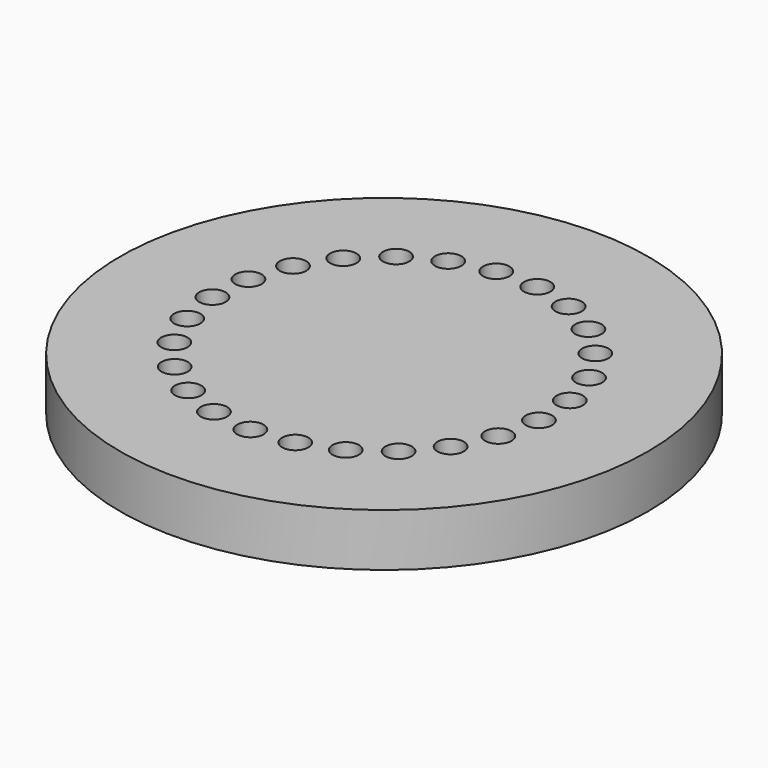
from build123d import *

# Parameters (mm, degrees)
F0_R     = 5080
F1_DEPTH = 508


# Not quite as in the source:
# - a feature names something its author has since deleted; it is built from what else it names


with BuildPart() as f1:
    # F0 (on Top) → F1 (new body, symmetric)
    with BuildSketch(Plane.XY):
        Circle(F0_R)
        with BuildLine():
            ThreePointArc((3159.7651539423, 310.6592537359), (3170.6487728458, 166.1666610714), (3174.9283642102, 21.3279659893))
            ThreePointArc((3174.9283642102, 21.3279659892), (3349.0433755669, -55.9407103788), (3420.4734651877, -232.5312758802))
            ThreePointArc((3420.4734651877, -232.5312758802), (3335.6199052673, -422.018694482), (3137.7531359879, -484.902317584))
            ThreePointArc((3137.7531359879, -484.902317584), (3112.360979424, -627.5620557037), (3080.486200819, -768.9146679337))
            ThreePointArc((3080.486200819, -768.9146679337), (3212.4276604766, -860.3797880933), (3263.1647017804, -1012.6958070214))
            ThreePointArc((3263.1647017804, -1012.6958070214), (3153.2283007654, -1221.8887310114), (2918.5845486504, -1249.9956929441))
            ThreePointArc((2918.5845486504, -1249.9956929442), (2858.512099202, -1381.8587405071), (2792.4857601946, -1510.8435653999))
            ThreePointArc((2792.4857601946, -1510.8435654), (2883.5294819577, -1603.5895784257), (2916.7790532267, -1729.2289361727))
            ThreePointArc((2916.7790532267, -1729.2289361727), (2779.4878421015, -1954.8282681739), (2516.0305603182, -1936.547241754))
            ThreePointArc((2516.0305603182, -1936.5472417539), (2425.052390915, -2049.3281585235), (2329.0231692129, -2157.8406051582))
            ThreePointArc((2329.0231692129, -2157.8406051582), (2383.8377363773, -2240.1269627642), (2403.0812037424, -2337.1082516052))
            ThreePointArc((2403.0812037424, -2337.1082516052), (2236.5946151881, -2575.5561553853), (1955.385118568, -2501.4184052418))
            ThreePointArc((1955.385118568, -2501.4184052419), (1839.217722188, -2588.0307514382), (1719.2194869615, -2669.2525837118))
            ThreePointArc((1719.2194869615, -2669.2525837117), (1745.4090642416, -2731.3446932303), (1754.3486784592, -2798.1384603063))
            ThreePointArc((1754.3486784592, -2798.1384603063), (1557.2865736992, -3045.674469981), (1271.8756384148, -2909.116250755))
            ThreePointArc((1271.8756384147, -2909.116250755), (1137.8182398063, -2964.1178541286), (1001.3909214974, -3012.9456056064))
            ThreePointArc((1001.3909214974, -3012.9456056064), (1008.843218066, -3047.7984710094), (1011.343727812, -3083.3513387131))
            ThreePointArc((1011.343727812, -3083.3513387131), (782.8081622254, -3336.0716635388), (508.4495342686, -3134.0236232521))
            ThreePointArc((508.4495342686, -3134.0236232521), (364.9254528148, -3153.9585307813), (220.6412815773, -3167.3241742619))
            ThreePointArc((220.6412815773, -3167.3241742619), (220.7243829568, -3171.0746343661), (220.7520854309, -3174.8259127355))
            ThreePointArc((220.7520854309, -3174.8259127355), (-39.6585303247, -3428.745002222), (-286.9243240623, -3162.0087653676))
            ThreePointArc((-286.9243240623, -3162.0087653676), (-430.8969424789, -3145.6243934968), (-573.972061526, -3122.6881164451))
            ThreePointArc((-573.9720615261, -3122.6881164451), (-887.4905056565, -3312.1596583452), (-1064.2696718785, -2991.3132677003))
            ThreePointArc((-1064.2696718784, -2991.3132677003), (-1199.6444981486, -2939.6391067717), (-1332.5206290822, -2881.8420798285))
            ThreePointArc((-1332.5206290822, -2881.8420798285), (-1683.3089711463, -2987.3921583311), (-1774.7430421005, -2632.6625561427))
            ThreePointArc((-1774.7430421005, -2632.6625561427), (-1893.0139780159, -2548.9454837318), (-2007.3420248451, -2459.9193066625))
            ThreePointArc((-2007.342024845, -2459.9193066625), (-2373.3589432016, -2474.9158221493), (-2373.702779939, -2108.5919739271))
            ThreePointArc((-2373.7027799391, -2108.591973927), (-2467.4384276259, -1998.0922415832), (-2556.0347386993, -1883.4307565086))
            ThreePointArc((-2556.0347386993, -1883.4307565086), (-2914.282044252, -1806.9314227581), (-2823.5140422458, -1452.0308031309))
            ThreePointArc((-2823.5140422458, -1452.0308031309), (-2886.8246462244, -1321.6915154268), (-2944.1223894829, -1188.5993251494))
            ThreePointArc((-2944.1223894829, -1188.5993251494), (-3272.0900864823, -1025.4108766461), (-3095.91353312, -704.2331967781))
            ThreePointArc((-3095.91353312, -704.2331967781), (-3124.8210553023, -562.2440505147), (-3147.2200028105, -419.0838268286))
            ThreePointArc((-3147.2200028105, -419.0838268285), (-3424.3006746734, -179.4599939571), (-3173.7853907348, 87.8139713167))
            ThreePointArc((-3173.7853907348, 87.8139713168), (-3166.4734651876, 232.5312758803), (-3152.5662086961, 376.7642496146))
            ThreePointArc((-3152.5662086961, 376.7642496145), (-3361.3498577779, 677.76702016), (-3052.2366398835, 874.3434646365))
            ThreePointArc((-3052.2366398835, 874.3434646365), (-3009.1647017804, 1012.6958070214), (-2959.8250853618, 1148.9388426122))
            ThreePointArc((-2959.8250853618, 1148.9388426122), (-3087.1930671381, 1492.4074397477), (-2738.9046356072, 1605.9347424628))
            ThreePointArc((-2738.9046356072, 1605.9347424629), (-2662.7790532267, 1729.2289361727), (-2581.107266439, 1848.9213826271))
            ThreePointArc((-2581.107266439, 1848.9213826271), (-2619.0565821882, 2213.2744112054), (-2253.4771800891, 2236.6192342054))
            ThreePointArc((-2253.4771800891, 2236.6192342054), (-2149.0812037424, 2337.1082516052), (-2040.2089853173, 2432.7293923144))
            ThreePointArc((-2040.2089853173, 2432.7293923144), (-1986.355139963, 2795.0732115532), (-1626.4554656367, 2726.7687137527))
            ThreePointArc((-1626.4554656367, 2726.7687137527), (-1500.3486784592, 2798.1384603064), (-1371.1168702844, 2863.6800673297))
            ThreePointArc((-1371.1168702844, 2863.6800673297), (-1228.8436989908, 3201.2472824589), (-897.2375725935, 3045.5852866611))
            ThreePointArc((-897.2375725935, 3045.5852866611), (-757.343727812, 3083.3513387131), (-615.8724396764, 3114.6951918361))
            ThreePointArc((-615.8724396764, 3114.6951918361), (-394.11948904, 3406.2752132438), (-111.6429430553, 3173.0365351294))
            ThreePointArc((-111.6429430552, 3173.0365351294), (33.2479145692, 3174.8259127355), (178.0695213369, 3170.0025623918))
            ThreePointArc((178.0695213369, 3170.0025623918), (443.1001189081, 3399.3310794258), (684.8969424789, 3145.6243934968))
            ThreePointArc((684.8969424789, 3145.6243934968), (683.9124547508, 3123.2827160797), (680.9666231891, 3101.1142284834))
            ThreePointArc((680.9666231891, 3101.1142284834), (821.7504682005, 3066.8144984678), (960.8227194307, 3026.1270134986))
            ThreePointArc((960.8227194307, 3026.1270134986), (1243.5493282112, 3189.815776142), (1453.6444981486, 2939.6391067717))
            ThreePointArc((1453.6444981486, 2939.6391067717), (1447.8647528602, 2885.7623478592), (1430.7885520784, 2834.3375097615))
            ThreePointArc((1430.7885520784, 2834.3375097615), (1558.619417728, 2766.1038503066), (1683.2038924038, 2692.1087750306))
            ThreePointArc((1683.2038924039, 2692.1087750306), (1967.9280563141, 2791.6467010191), (2147.0139780158, 2548.9454837318))
            ThreePointArc((2147.0139780158, 2548.9454837318), (2132.5243934708, 2464.3833119964), (2090.7087741685, 2389.4689413371))
            ThreePointArc((2090.7087741685, 2389.4689413372), (2197.5545770385, 2291.5887242123), (2299.8231744264, 2188.9354413438))
            ThreePointArc((2299.8231744264, 2188.9354413439), (2572.1803143936, 2229.4904636082), (2721.4384276259, 1998.0922415832))
            ThreePointArc((2721.4384276259, 1998.0922415832), (2694.4617814958, 1884.1782529882), (2619.2620748886, 1794.4612514765))
            ThreePointArc((2619.2620748885, 1794.4612514766), (2698.4093002333, 1673.084650702), (2771.9361082418, 1548.2232435361))
            ThreePointArc((2771.9361082418, 1548.2232435361), (3019.7424993376, 1538.1374539976), (3140.8246462244, 1321.6915154268))
            ThreePointArc((3140.8246462244, 1321.6915154268), (3097.7806446017, 1180.2222016211), (2983.2375064713, 1086.7009616187))
            ThreePointArc((2983.2375064713, 1086.7009616187), (3029.7130430392, 949.4545154131), (3069.8781019084, 810.2304853702))
            ThreePointArc((3069.8781019084, 810.2304853702), (3283.818680816, 760.3242238815), (3378.8210553023, 562.2440505147))
            ThreePointArc((3378.8210553023, 562.2440505147), (3316.3827960735, 395.4504670868), (3159.7651539423, 310.6592537359))
        make_face(mode=Mode.SUBTRACT)
        with BuildLine():
            ThreePointArc((3137.7531359879, -484.902317584), (2913.1555879726, -213.9287738098), (3174.9283642102, 21.3279659892))
            ThreePointArc((3174.9283642102, 21.3279659893), (3170.6487728458, 166.1666610714), (3159.7651539423, 310.6592537359))
            ThreePointArc((3159.7651539423, 310.6592537359), (2874.8353708782, 517.2645264735), (3069.8781019084, 810.2304853702))
            ThreePointArc((3069.8781019084, 810.2304853702), (3029.7130430392, 949.4545154131), (2983.2375064713, 1086.7009616187))
            ThreePointArc((2983.2375064713, 1086.7009616187), (2655.8786745265, 1215.9561941926), (2771.9361082418, 1548.2232435361))
            ThreePointArc((2771.9361082418, 1548.2232435361), (2698.4093002333, 1673.084650702), (2619.2620748885, 1794.4612514766))
            ThreePointArc((2619.2620748886, 1794.4612514765), (2270.0433534158, 1838.2448622566), (2299.8231744264, 2188.9354413439))
            ThreePointArc((2299.8231744264, 2188.9354413438), (2197.5545770385, 2291.5887242123), (2090.7087741685, 2389.4689413372))
            ThreePointArc((2090.7087741685, 2389.4689413371), (1741.5728597746, 2345.0298450332), (1683.2038924039, 2692.1087750306))
            ThreePointArc((1683.2038924038, 2692.1087750306), (1558.619417728, 2766.1038503066), (1430.7885520784, 2834.3375097615))
            ThreePointArc((1430.7885520784, 2834.3375097615), (1103.6729382967, 2704.46797823), (960.8227194307, 3026.1270134986))
            ThreePointArc((960.8227194307, 3026.1270134986), (821.7504682005, 3066.8144984678), (680.9666231891, 3101.1142284834))
            ThreePointArc((680.9666231891, 3101.1142284834), (396.4251870806, 2893.9744420171), (178.0695213369, 3170.0025623918))
            ThreePointArc((178.0695213369, 3170.0025623918), (33.2479145692, 3174.8259127355), (-111.6429430552, 3173.0365351294))
            ThreePointArc((-111.6429430553, 3173.0365351294), (-111.1048887554, 3163.5042764587), (-110.9254528149, 3153.9585307813))
            ThreePointArc((-110.9254528149, 3153.9585307813), (-345.2345242287, 2900.7229342878), (-615.8724396764, 3114.6951918361))
            ThreePointArc((-615.8724396764, 3114.6951918361), (-757.343727812, 3083.3513387131), (-897.2375725935, 3045.5852866611))
            ThreePointArc((-897.2375725935, 3045.5852866611), (-887.1955258795, 3005.4004807889), (-883.8182398063, 2964.1178541286))
            ThreePointArc((-883.8182398063, 2964.1178541286), (-1086.5437439113, 2715.3470237029), (-1371.1168702844, 2863.6800673297))
            ThreePointArc((-1371.1168702844, 2863.6800673297), (-1500.3486784592, 2798.1384603064), (-1626.4554656367, 2726.7687137527))
            ThreePointArc((-1626.4554656367, 2726.7687137527), (-1595.7453283073, 2660.3992073978), (-1585.217722188, 2588.0307514382))
            ThreePointArc((-1585.217722188, 2588.0307514382), (-1757.1682884144, 2347.6479516845), (-2040.2089853173, 2432.7293923144))
            ThreePointArc((-2040.2089853173, 2432.7293923144), (-2149.0812037424, 2337.1082516052), (-2253.4771800891, 2236.6192342054))
            ThreePointArc((-2253.4771800891, 2236.6192342054), (-2192.5700221752, 2151.6411500012), (-2171.052390915, 2049.3281585235))
            ThreePointArc((-2171.052390915, 2049.3281585235), (-2313.5219878473, 1821.1243697917), (-2581.107266439, 1848.9213826271))
            ThreePointArc((-2581.107266439, 1848.9213826271), (-2662.7790532267, 1729.2289361727), (-2738.9046356072, 1605.9347424629))
            ThreePointArc((-2738.9046356072, 1605.9347424628), (-2640.6861414363, 1512.5027305085), (-2604.512099202, 1381.8587405071))
            ThreePointArc((-2604.512099202, 1381.8587405071), (-2719.2596279216, 1169.4328728679), (-2959.8250853618, 1148.9388426122))
            ThreePointArc((-2959.8250853618, 1148.9388426122), (-3009.1647017804, 1012.6958070214), (-3052.2366398835, 874.3434646365))
            ThreePointArc((-3052.2366398835, 874.3434646365), (-2912.6266781094, 784.4767104635), (-2858.360979424, 627.5620557037))
            ThreePointArc((-2858.360979424, 627.5620557037), (-2947.5825345884, 434.2641919867), (-3152.5662086961, 376.7642496145))
            ThreePointArc((-3152.5662086961, 376.7642496146), (-3166.4734651876, 232.5312758803), (-3173.7853907348, 87.8139713168))
            ThreePointArc((-3173.7853907348, 87.8139713167), (-2992.1560572294, 14.5440206049), (-2916.6487728458, -166.1666610713))
            ThreePointArc((-2916.6487728458, -166.1666610713), (-2982.9430089639, -337.2880980847), (-3147.2200028105, -419.0838268285))
            ThreePointArc((-3147.2200028105, -419.0838268286), (-3124.8210553023, -562.2440505147), (-3095.91353312, -704.2331967781))
            ThreePointArc((-3095.91353312, -704.2331967781), (-2875.2768498728, -747.7977222216), (-2775.7130430392, -949.4545154131))
            ThreePointArc((-2775.7130430392, -949.4545154131), (-2822.0401921375, -1095.7008384381), (-2944.1223894829, -1188.5993251494))
            ThreePointArc((-2944.1223894829, -1188.5993251494), (-2886.8246462244, -1321.6915154268), (-2823.5140422458, -1452.0308031309))
            ThreePointArc((-2823.5140422458, -1452.0308031309), (-2570.4651805387, -1453.6619940879), (-2444.4093002333, -1673.084650702))
            ThreePointArc((-2444.4093002333, -1673.084650702), (-2474.0444872282, -1792.1494678613), (-2556.0347386993, -1883.4307565086))
            ThreePointArc((-2556.0347386993, -1883.4307565086), (-2467.4384276259, -1998.0922415832), (-2373.7027799391, -2108.591973927))
            ThreePointArc((-2373.702779939, -2108.5919739271), (-2098.1202860136, -2057.8606305471), (-1943.5545770385, -2291.5887242123))
            ThreePointArc((-1943.5545770385, -2291.5887242123), (-1960.0361690602, -2381.5943122134), (-2007.342024845, -2459.9193066625))
            ThreePointArc((-2007.3420248451, -2459.9193066625), (-1893.0139780159, -2548.9454837318), (-1774.7430421005, -2632.6625561427))
            ThreePointArc((-1774.7430421005, -2632.6625561427), (-1489.2630935413, -2521.7563512498), (-1304.6194177281, -2766.1038503066))
            ThreePointArc((-1304.6194177281, -2766.1038503066), (-1311.6932219569, -2825.63076726), (-1332.5206290822, -2881.8420798285))
            ThreePointArc((-1332.5206290822, -2881.8420798285), (-1199.6444981486, -2939.6391067717), (-1064.2696718784, -2991.3132677003))
            ThreePointArc((-1064.2696718785, -2991.3132677003), (-783.5659015158, -2815.7011000457), (-567.7504682005, -3066.8144984678))
            ThreePointArc((-567.7504682005, -3066.8144984678), (-569.3106582504, -3094.9239693334), (-573.9720615261, -3122.6881164451))
            ThreePointArc((-573.972061526, -3122.6881164451), (-430.8969424789, -3145.6243934968), (-286.9243240623, -3162.0087653676))
            ThreePointArc((-286.9243240623, -3162.0087653676), (-30.5880814035, -2920.8398397167), (220.6412815773, -3167.3241742619))
            ThreePointArc((220.6412815773, -3167.3241742619), (364.9254528148, -3153.9585307813), (508.4495342686, -3134.0236232521))
            ThreePointArc((508.4495342686, -3134.0236232521), (696.756229587, -2836.683231616), (1001.3909214974, -3012.9456056064))
            ThreePointArc((1001.3909214974, -3012.9456056064), (1137.8182398063, -2964.1178541286), (1271.8756384147, -2909.116250755))
            ThreePointArc((1271.8756384148, -2909.116250755), (1380.3207841825, -2574.2873834818), (1719.2194869615, -2669.2525837117))
            ThreePointArc((1719.2194869615, -2669.2525837118), (1839.217722188, -2588.0307514382), (1955.385118568, -2501.4184052419))
            ThreePointArc((1955.385118568, -2501.4184052418), (1977.1547074431, -2150.1395914767), (2329.0231692129, -2157.8406051582))
            ThreePointArc((2329.0231692129, -2157.8406051582), (2425.052390915, -2049.3281585235), (2516.0305603182, -1936.5472417539))
            ThreePointArc((2516.0305603182, -1936.547241754), (2449.7567289686, -1590.8906212789), (2792.4857601946, -1510.8435654))
            ThreePointArc((2792.4857601946, -1510.8435653999), (2858.512099202, -1381.8587405071), (2918.5845486504, -1249.9956929442))
            ThreePointArc((2918.5845486504, -1249.9956929441), (2768.431525638, -931.6801424597), (3080.486200819, -768.9146679337))
            ThreePointArc((3080.486200819, -768.9146679337), (3112.360979424, -627.5620557037), (3137.7531359879, -484.902317584))
        make_face()
    extrude(amount=F1_DEPTH, both=True)


solid = f1.part
